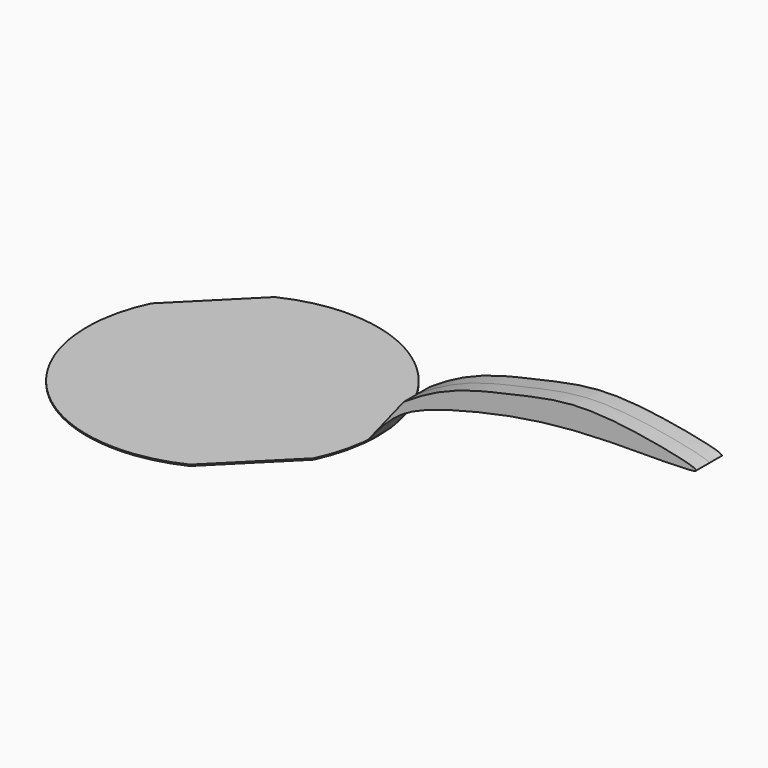
from build123d import *

# Parameters (mm, degrees)
F4_DEPTH = 0.508
F6_DEPTH = 6.35


# Not quite as in the source:
# - the program builds the solid bodies; features that only make, move or delete a surface that nothing else refers to are left out


with BuildPart() as f4:
    # F0 (on Top) → F4 (new body)
    with BuildSketch(Plane.XY):
        with BuildLine():
            Line((-6.0308964237, -56.8308964237), (56.8308964237, 6.0308964237))
            ThreePointArc((56.8308964237, 6.0308964237), (56.009443014, 11.3606686977), (54.689286609, 16.589286609))
            Line((54.689286609, 16.589286609), (-16.589286609, -54.689286609))
            ThreePointArc((-16.589286609, -54.689286609), (-11.3606686977, -56.009443014), (-6.0308964237, -56.8308964237))
        make_face()
        with BuildLine():
            Line((-16.589286609, -54.689286609), (54.689286609, 16.589286609))
            ThreePointArc((54.689286609, 16.589286609), (53.0707840703, 21.2041122936), (51.0636709662, 25.6636709662))
            Line((51.0636709662, 25.6636709662), (-25.6636709662, -51.0636709662))
            ThreePointArc((-25.6636709662, -51.0636709662), (-21.2041122936, -53.0707840703), (-16.589286609, -54.689286609))
        make_face()
        with BuildLine():
            Line((-25.6636709662, -51.0636709662), (51.0636709662, 25.6636709662))
            ThreePointArc((51.0636709662, 25.6636709662), (48.8212712491, 29.7086851548), (46.2591311607, 33.5591311607))
            Line((46.2591311607, 33.5591311607), (-33.5591311607, -46.2591311607))
            ThreePointArc((-33.5591311607, -46.2591311607), (-29.7086851548, -48.8212712491), (-25.6636709662, -51.0636709662))
        make_face()
        with BuildLine():
            Line((-33.5591311607, -46.2591311607), (46.2591311607, 33.5591311607))
            ThreePointArc((46.2591311607, 33.5591311607), (43.4703585062, 37.1005448928), (40.4111525448, 40.4111525448))
            Line((40.4111525448, 40.4111525448), (-40.4111525448, -40.4111525448))
            ThreePointArc((-40.4111525448, -40.4111525448), (-37.1005448928, -43.4703585062), (-33.5591311607, -46.2591311607))
        make_face()
        with BuildLine():
            Line((-40.4111525448, -40.4111525448), (40.4111525448, 40.4111525448))
            ThreePointArc((40.4111525448, 40.4111525448), (37.1005448928, 43.4703585062), (33.5591311607, 46.2591311607))
            Line((33.5591311607, 46.2591311607), (-46.2591311607, -33.5591311607))
            ThreePointArc((-46.2591311607, -33.5591311607), (-43.4703585062, -37.1005448928), (-40.4111525448, -40.4111525448))
        make_face()
        with BuildLine():
            Line((-46.2591311607, -33.5591311607), (33.5591311607, 46.2591311607))
            ThreePointArc((33.5591311607, 46.2591311607), (29.7086851548, 48.8212712491), (25.6636709662, 51.0636709662))
            Line((25.6636709662, 51.0636709662), (-51.0636709662, -25.6636709662))
            ThreePointArc((-51.0636709662, -25.6636709662), (-48.8212712491, -29.7086851548), (-46.2591311607, -33.5591311607))
        make_face()
        with BuildLine():
            Line((-51.0636709662, -25.6636709662), (25.6636709662, 51.0636709662))
            ThreePointArc((25.6636709662, 51.0636709662), (21.2041122936, 53.0707840703), (16.589286609, 54.689286609))
            Line((16.589286609, 54.689286609), (-54.689286609, -16.589286609))
            ThreePointArc((-54.689286609, -16.589286609), (-53.0707840703, -21.2041122936), (-51.0636709662, -25.6636709662))
        make_face()
        with BuildLine():
            Line((-54.689286609, -16.589286609), (16.589286609, 54.689286609))
            ThreePointArc((16.589286609, 54.689286609), (11.3606686977, 56.009443014), (6.0308964237, 56.8308964237))
            Line((6.0308964237, 56.8308964237), (-56.8308964237, -6.0308964237))
            ThreePointArc((-56.8308964237, -6.0308964237), (-56.009443014, -11.3606686977), (-54.689286609, -16.589286609))
        make_face()
        with BuildLine():
            Line((-56.8308964237, -6.0308964237), (6.0308964237, 56.8308964237))
            ThreePointArc((6.0308964237, 56.8308964237), (-0.3618335895, 57.1488545507), (-6.750025, 56.749975))
            Line((-6.750025, 56.749975), (-56.749975, 6.750025))
            ThreePointArc((-56.749975, 6.750025), (-57.1488545507, 0.3618335895), (-56.8308964237, -6.0308964237))
        make_face()
        with BuildLine():
            Line((-56.749975, 6.750025), (-6.750025, 56.749975))
            ThreePointArc((-6.750025, 56.749975), (-15.9021226487, 54.8930323016), (-24.6296158184, 51.5703841816))
            Line((-24.6296158184, 51.5703841816), (-51.5703841816, 24.6296158184))
            ThreePointArc((-51.5703841816, 24.6296158184), (-54.8930323016, 15.9021226487), (-56.749975, 6.750025))
        make_face()
        with BuildLine():
            ThreePointArc((56.749975, -6.750025), (57.0499060965, -3.3809339502), (57.15, 0))
            ThreePointArc((57.15, 0), (57.0701683483, 3.0196663212), (56.8308964237, 6.0308964237))
            Line((56.8308964237, 6.0308964237), (-6.0308964237, -56.8308964237))
            ThreePointArc((-6.0308964237, -56.8308964237), (0.3618335895, -57.1488545507), (6.750025, -56.749975))
            Line((6.750025, -56.749975), (56.749975, -6.750025))
        make_face()
        with BuildLine():
            ThreePointArc((51.5703841816, -24.6296158184), (54.8930323016, -15.9021226487), (56.749975, -6.750025))
            Line((56.749975, -6.750025), (6.750025, -56.749975))
            ThreePointArc((6.750025, -56.749975), (15.9021226487, -54.8930323016), (24.6296158184, -51.5703841816))
            Line((24.6296158184, -51.5703841816), (51.5703841816, -24.6296158184))
        make_face()
    extrude(amount=-F4_DEPTH)


with BuildPart() as f6:
    # F5 (on Front) → F6 (new body, symmetric)
    with BuildSketch(Plane.XZ):
        with BuildLine():
            Line((72.3931133133, 18.8288400268), (57.4625453009, 0))
            add(Edge.make_bspline(
                [(57.4625453009, 0), (60.0150991548, 3.025146449), (64.4408409242, 8.6698817024), (74.6149706503, 17.3720244011), (99.8845177525, 24.9056378613), (139.8560927381, 33.0040594631), (205.2990521286, 30.1110742823), (158.0984786426, 39.5886639029), (134.9190645718, 40.0712558659), (110.2767996195, 34.0103979924), (87.8425301448, 29.4073637277), (72.3931133133, 18.8288400268)],
                knots=[0, 0, 0, 0, 0.0708652491, 0.1462220586, 0.2516287369, 0.400965123, 0.537935388, 0.6471743961, 0.7586724699, 0.860910477, 1, 1, 1, 1], degree=3))
        make_face()
    extrude(amount=F6_DEPTH, both=True)


solid = Compound([f4.part, f6.part])
